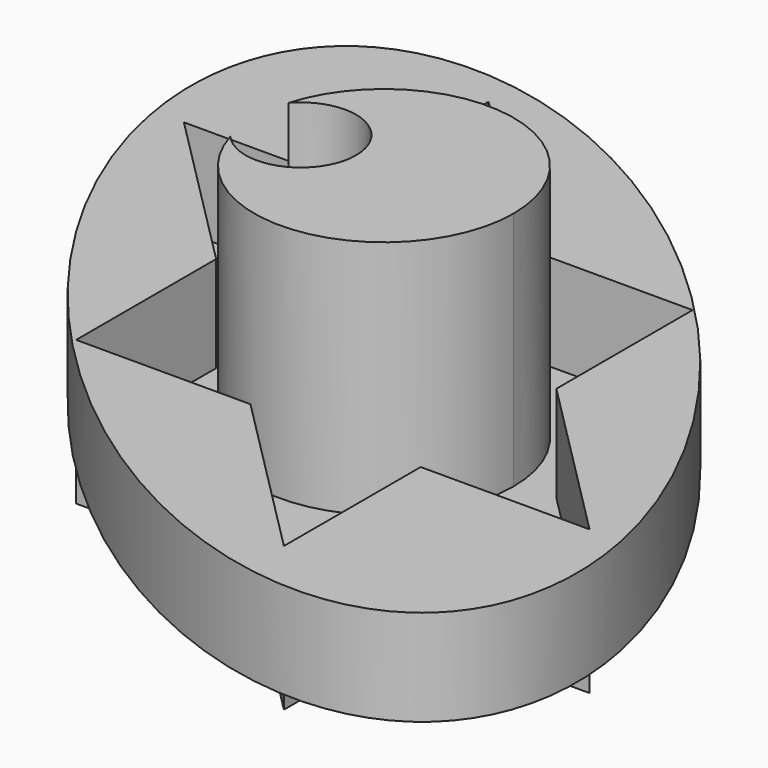
from build123d import *

# Parameters (mm, degrees)
F1_DEPTH     = 5
F3_DEPTH     = 10
F4_TEXT_SIZE = 13.4309564893
F5_DEPTH     = 1
F7_DEPTH     = 25


# Not quite as in the source:
# - Text() gives the source's letters only with a copy of the font that has no kerning and outlines rounded to 1/6400 em; it was checked with that copy


with BuildPart() as f1:
    # F0 (on Top) → F1 (new body)
    with BuildSketch(Plane.XY):
        Polygon((-18.3897209494, 18.3052610722), (-18.3834756345, 1.1537321024), (-0.2460259832, -17.0593304155), (17.4649701775, -17.0505742449), (17.4649701775, 0.5935830002), (-0.1797797445, 18.3118917824), align=None)
        Polygon((-0.2460259832, -17.0593304155), (-18.3834756345, 1.1537321024), (-18.3768405238, -17.0682941409), align=None)
        Polygon((17.4649701775, -17.0505742449), (-0.2460259832, -17.0593304155), (17.4649701775, -34.8441616091), align=None)
        Polygon((17.4649701775, 0.5935830002), (17.4649701775, -17.0505742449), (35.027229818, -17.0418916083), align=None)
        Polygon((-18.3897209494, 18.3052610722), (-35.4576097142, 18.2990462128), (-18.3834756345, 1.1537321024), align=None)
        Polygon((17.4649701775, 18.3183166918), (-0.1797797445, 18.3118917824), (17.4649701775, 0.5935830002), align=None)
        Polygon((-18.396384153, 36.6044390443), (-18.3897209494, 18.3052610722), (-0.1797797445, 18.3118917824), align=None)
    extrude(amount=F1_DEPTH)

    # F4 (on face) → F5 (join)
    with BuildSketch(Plane(origin=(0, 0, 0), x_dir=(1, 0, 0), z_dir=(0, 0, -1))):
        with Locations(Location((-13.7695586141, -20.1421609659), (0, 0, 44.5986286526))):
            Text('danger', F4_TEXT_SIZE, font='Open Sans', text_align=(TextAlign.LEFT, TextAlign.BOTTOM))
    extrude(amount=F5_DEPTH)

    # F6 (on face) → F7 (join)
    with BuildSketch(Plane.XY.offset(5)):
        with BuildLine():
            ThreePointArc((-12.9485539481, 3.7968127201), (-6.6167093231, 5.3670909715), (-2.9082912446, 0))
            ThreePointArc((-2.9082912446, 0), (-6.6167093231, -5.3670909715), (-12.9485539481, -3.7968127201))
            ThreePointArc((-12.9485539481, -3.7968127201), (1.9178769036, -13.3567430297), (13.4937332188, 0))
            ThreePointArc((13.4937332188, 0), (1.9178769036, 13.3567430297), (-12.9485539481, 3.7968127201))
        make_face()
    extrude(amount=F7_DEPTH)


with BuildPart() as f3:
    # F2 (on face) → F3 (new body)
    with BuildSketch(Plane.XY.offset(5)):
        with BuildLine():
            add(Edge.make_bspline(
                [(34.3890926731, -36.2958717366), (66.392512019, -5.9737303722), (-1.1928366636, 33.3090065505), (-68.7781853461, 72.5917434733), (-33.1962560095, 2.9868651861), (2.3856733271, -66.6180131011), (34.3890926731, -36.2958717366)],
                knots=[0, 0, 0, 2.0943951024, 2.0943951024, 4.1887902048, 4.1887902048, 6.2831853072, 6.2831853072, 6.2831853072], degree=2, weights=[1, 0.5, 1, 0.5, 1, 0.5, 1]))
        make_face()
        Polygon((-18.3768405238, -17.0682941409), (-18.3834756345, 1.1537321024), (-35.4576097142, 18.2990462128), (-18.3897209494, 18.3052610722), (-18.396384153, 36.6044390443), (-0.1797797445, 18.3118917824), (17.4649701775, 18.3183166918), (17.4649701775, 0.5935830002), (35.027229818, -17.0418916083), (17.4649701775, -17.0505742449), (17.4649701775, -34.8441616091), (-0.2460259832, -17.0593304155), align=None, mode=Mode.SUBTRACT)
    extrude(amount=F3_DEPTH)


solid = Compound([f1.part, f3.part])
